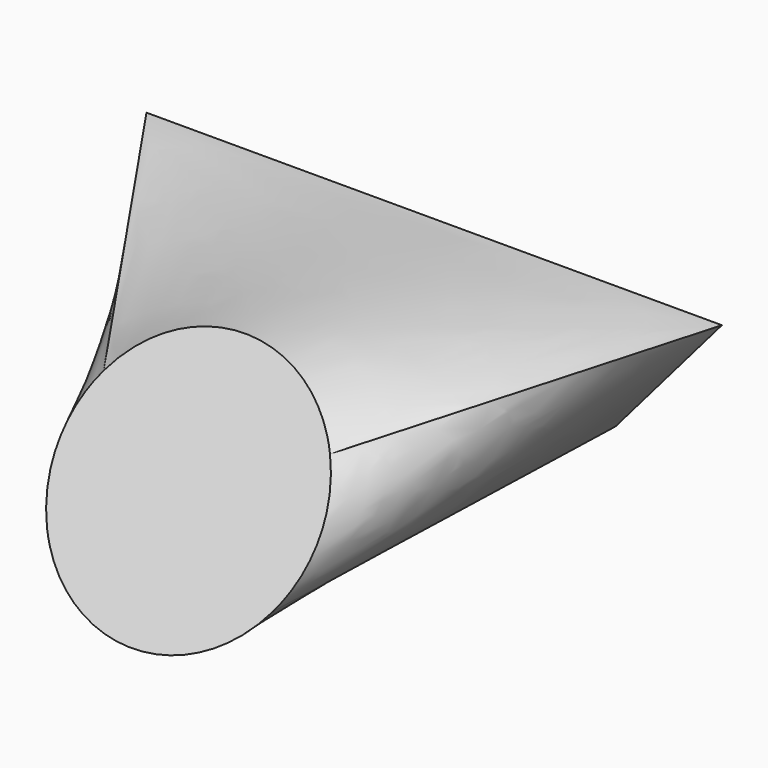
from build123d import *


# Not quite as in the source:
# - the arcs of a loft's sections are written as splines that run evenly, so that the points pair up as in the source's solid


with BuildPart() as f4:
    # F0 (on Front) → F4 section 0
    with BuildSketch(Plane.XZ):
        Polygon((58.8329508901, 13.2794305682), (0, 13.2794305682), (-58.8329508901, 13.2794305682), (-37.0616838336, -12.0401540771), (0, -12.0401540771), (37.0616838336, -12.0401540771), align=None)
    # F3 (on face) → F4 section 1
    with BuildSketch(Plane(origin=(0, -39.5994907451, 25.6573906524), x_dir=(-1, 0, 0), z_dir=(0, 0.8392395084, -0.5437619402))):
        with BuildLine():
            add(Edge.make_bspline(
                [(0, -15.9545506842), (-1.5537470677, -15.9545506842), (-3.107470141, -16.0904838393), (-6.167754458, -16.6300945331), (-7.674268442, -17.0337637385), (-10.5943577501, -18.096589328), (-12.0078879796, -18.7557292991), (-14.699056843, -20.3094763668), (-15.9766539173, -21.204059469), (-18.3571325318, -23.2015181964), (-19.4599773103, -24.304362975), (-21.4574360377, -26.6848415894), (-22.35201914, -27.9624386638), (-23.1288926738, -29.3080230955)],
                knots=[0, 0, 0, 0, 0.1666666667, 0.1666666667, 0.3333333333, 0.3333333333, 0.5, 0.5, 0.6666666667, 0.6666666667, 0.8333333333, 0.8333333333, 1, 1, 1, 1], degree=3))
            add(Edge.make_bspline(
                [(-23.1288926738, -29.3080230955), (-23.9057662077, -30.6536075271), (-24.5649061788, -32.0671377567), (-25.6277317683, -34.9872270648), (-26.0314009737, -36.4937410488), (-26.5710116674, -39.5540253657), (-26.7069448226, -41.1077484391), (-26.7069448226, -44.2152425744), (-26.5710116674, -45.7689656478), (-26.0314009737, -48.8292499647), (-25.6277317683, -50.3357639487), (-24.5649061788, -53.2558532568), (-23.9057662077, -54.6693834864), (-23.1288926738, -56.0149679181)],
                knots=[0, 0, 0, 0, 0.1666666667, 0.1666666667, 0.3333333333, 0.3333333333, 0.5, 0.5, 0.6666666667, 0.6666666667, 0.8333333333, 0.8333333333, 1, 1, 1, 1], degree=3))
            add(Edge.make_bspline(
                [(-23.1288926738, -56.0149679181), (-22.35201914, -57.3605523497), (-21.4574360377, -58.6381494241), (-19.4599773103, -61.0186280385), (-18.3571325318, -62.1214728171), (-15.9766539173, -64.1189315445), (-14.699056843, -65.0135146468), (-12.0078879796, -66.5672617144), (-10.5943577501, -67.2264016855), (-7.674268442, -68.2892272751), (-6.167754458, -68.6928964805), (-3.107470141, -69.2325071742), (-1.5537470677, -69.3684403294), (0, -69.3684403294)],
                knots=[0, 0, 0, 0, 0.1666666667, 0.1666666667, 0.3333333333, 0.3333333333, 0.5, 0.5, 0.6666666667, 0.6666666667, 0.8333333333, 0.8333333333, 1, 1, 1, 1], degree=3))
            add(Edge.make_bspline(
                [(0, -69.3684403294), (1.5537470677, -69.3684403294), (3.107470141, -69.2325071742), (6.167754458, -68.6928964805), (7.674268442, -68.2892272751), (10.5943577501, -67.2264016855), (12.0078879796, -66.5672617144), (14.699056843, -65.0135146468), (15.9766539173, -64.1189315445), (18.3571325318, -62.1214728171), (19.4599773103, -61.0186280385), (21.4574360377, -58.6381494241), (22.35201914, -57.3605523497), (23.1288926738, -56.0149679181)],
                knots=[0, 0, 0, 0, 0.1666666667, 0.1666666667, 0.3333333333, 0.3333333333, 0.5, 0.5, 0.6666666667, 0.6666666667, 0.8333333333, 0.8333333333, 1, 1, 1, 1], degree=3))
            add(Edge.make_bspline(
                [(23.1288926738, -56.0149679181), (23.9057662077, -54.6693834864), (24.5649061788, -53.2558532568), (25.6277317683, -50.3357639487), (26.0314009737, -48.8292499647), (26.5710116674, -45.7689656478), (26.7069448226, -44.2152425744), (26.7069448226, -41.1077484391), (26.5710116674, -39.5540253657), (26.0314009737, -36.4937410488), (25.6277317683, -34.9872270648), (24.5649061788, -32.0671377567), (23.9057662077, -30.6536075271), (23.1288926738, -29.3080230955)],
                knots=[0, 0, 0, 0, 0.1666666667, 0.1666666667, 0.3333333333, 0.3333333333, 0.5, 0.5, 0.6666666667, 0.6666666667, 0.8333333333, 0.8333333333, 1, 1, 1, 1], degree=3))
            add(Edge.make_bspline(
                [(23.1288926738, -29.3080230955), (22.35201914, -27.9624386638), (21.4574360377, -26.6848415894), (19.4599773103, -24.304362975), (18.3571325318, -23.2015181964), (15.9766539173, -21.204059469), (14.699056843, -20.3094763668), (12.0078879796, -18.7557292991), (10.5943577501, -18.096589328), (7.674268442, -17.0337637385), (6.167754458, -16.6300945331), (3.107470141, -16.0904838393), (1.5537470677, -15.9545506842), (0, -15.9545506842)],
                knots=[0, 0, 0, 0, 0.1666666667, 0.1666666667, 0.3333333333, 0.3333333333, 0.5, 0.5, 0.6666666667, 0.6666666667, 0.8333333333, 0.8333333333, 1, 1, 1, 1], degree=3))
        make_face()
    loft(ruled=True)


solid = f4.part
